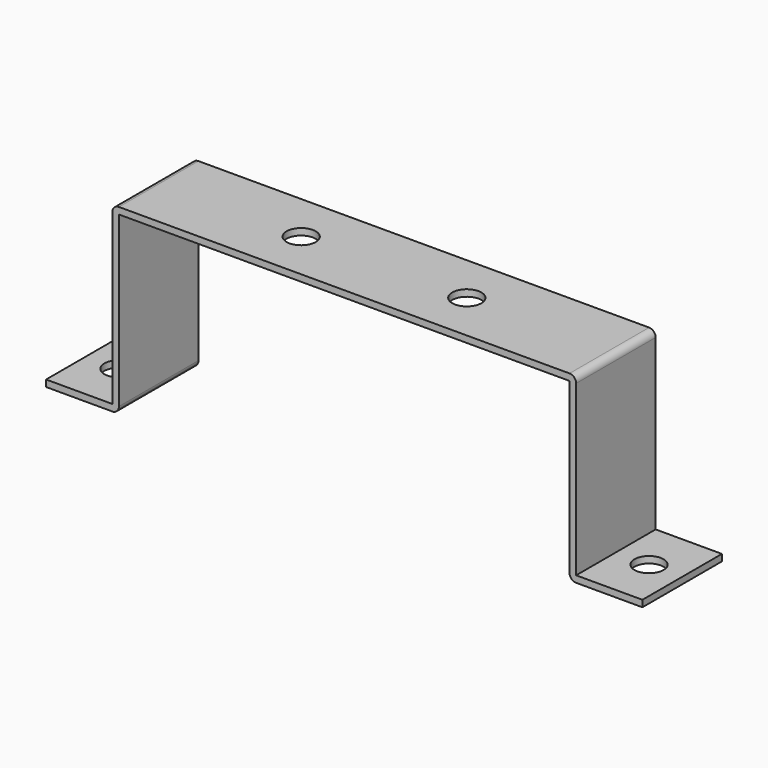
from build123d import *

# Parameters (mm, degrees)
F1_DEPTH = 30
F2_R     = 4.4
F3_R     = 4.4
F4_DEPTH = 25
F5_R     = 2
F6_R     = 2


# Not quite as in the source:
# - a feature names something its author has since deleted; it is built from what else it names


with BuildPart() as f1:
    # F0 (on Front) → F1 (new body)
    with BuildSketch(Plane.XZ):
        Polygon((90, -1), (90, 1), (70, 1), (70, 54), (-70, 54), (-70, 1), (-90, 1), (-90, -1), (-68, -1), (-68, 52), (68, 52), (68, -1), align=None)
    extrude(amount=F1_DEPTH)

    # F2 (on face) + F3 (on face) → F4 (cut)
    with BuildSketch(Plane.XY.offset(1)):
        with Locations((-80, -15)):
            Circle(F2_R)
        with Locations((80, -15)):
            Circle(F2_R)
    with BuildSketch(Plane.XY.offset(54)):
        with Locations((-25, -15)):
            Circle(F3_R)
        with Locations((25, -15)):
            Circle(F3_R)
    extrude(amount=-F4_DEPTH, mode=Mode.SUBTRACT)

    # F5
    f5_edges = [f1.edges().sort_by_distance(p)[0] for p in [
        (-70, -15, 54),
        (70, -15, 54),
    ]]
    fillet(f5_edges, radius=F5_R)

    # F6
    f6_edges = [f1.edges().sort_by_distance(p)[0] for p in [
        (68, -15, -1),
        (-68, -15, -1),
    ]]
    fillet(f6_edges, radius=F6_R)


solid = f1.part
